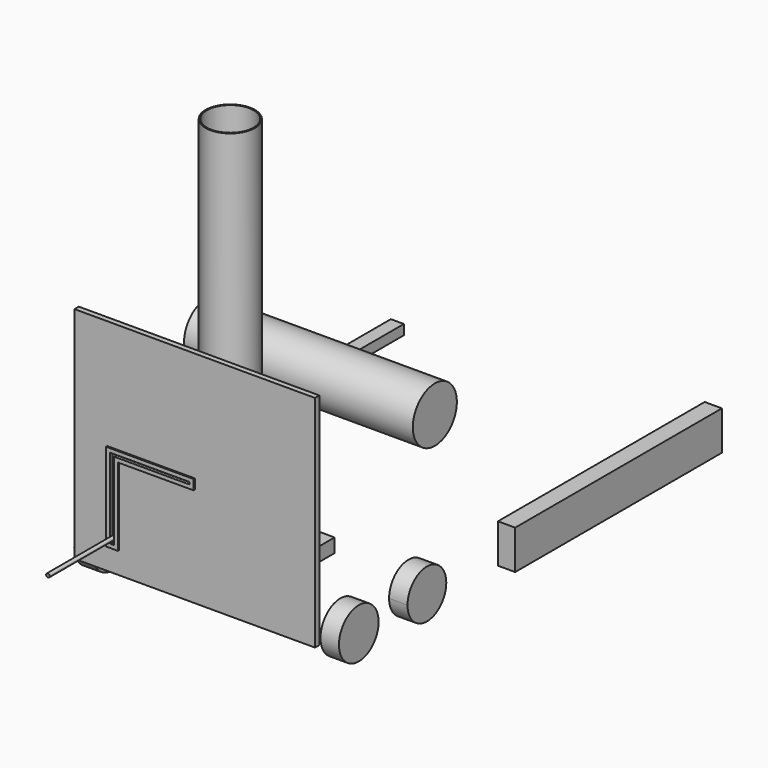
from build123d import *

# Parameters (mm, degrees)
F0_W      = 159.1055989265
F0_H      = 145.3896015882
F1_DEPTH  = 3.556
F6_R      = 18.1959049568
F7_DEPTH  = 151.384
F13_W     = 12.8093321323
F13_H     = 6.5816342831
F14_DEPTH = 36.068
F15_W     = 8.6199865751
F15_H     = 6.5816342831
F16_DEPTH = 170.942
F18_R     = 9.8295044078
F19_DEPTH = 25.4
F20_R     = 9.9402572171
F21_DEPTH = 1.016
F24_W     = 11.3966075535
F24_H     = 6.826877594
F25_DEPTH = 170.942
F26_R     = 16.3014838399
F27_DEPTH = 242.316
F28_R     = 15.4963138216
F29_DEPTH = 245.872
F31_DEPTH = 12.192
F33_DEPTH = 12.192
F34_W     = 34.9631672725
F34_H     = 28.9866179228
F35_DEPTH = 9.144
F36_T     = -2.54
F37_R     = 12.8059007853
F38_DEPTH = 3.048
F39_W     = 11.3966075535
F39_H     = 170.942
F40_DEPTH = 19.05
F43_W     = 50.1206144691
F43_H     = 6.5812724642
F44_DEPTH = 1.016
F45_T     = -2.54
F46_R     = 1.2184903026
F47_DEPTH = 54.864


# Not quite as in the source:
# - the program builds the solid bodies; features that only make, move or delete a surface that nothing else refers to are left out


with BuildPart() as f1:
    # F0 (on Front) → F1 (new body)
    with BuildSketch(Plane.XZ):
        Rectangle(F0_W, F0_H)
    extrude(amount=F1_DEPTH)

    # F18 (on face) → F19 (cut)
    with BuildSketch(Plane.XZ.offset(3.556)):
        with Locations((39.1956530511, -18.7452007085)):
            Circle(F18_R)
    extrude(amount=-F19_DEPTH, mode=Mode.SUBTRACT)

    # F20 (on face) → F21 (join)
    with BuildSketch(Plane.XZ.offset(3.556)):
        with Locations((39.1956530511, -18.7452007085)):
            Circle(F20_R)
    extrude(amount=-F21_DEPTH)

    # F43 (on face) → F44 (join)
    with BuildSketch(Plane.XZ.offset(3.556)):
        Polygon((-57.8088574111, 0), (-57.8088574111, -58.0925121903), (-50.1206144691, -58.0925121903), (-50.1206144691, -6.5812724642), (-50.1206144691, 0), align=None)
        with Locations((-25.0603072345, -3.2906362321)):
            Rectangle(F43_W, F43_H)
    extrude(amount=F44_DEPTH)

    # F45
    f45_openings = [f1.faces().sort_by_distance(p)[0] for p in [
        (-56.989309, -4.572, -29.046256),
    ]]
    offset(amount=F45_T, openings=f45_openings, kind=Kind.INTERSECTION)

    # F46 (on face) → F47 (join)
    with BuildSketch(Plane.XZ.offset(2.54)):
        with Locations((-54.0543831885, -52.2309578955)):
            Circle(F46_R)
    extrude(amount=F47_DEPTH)


with BuildPart() as f7:
    # F6 (on face) → F7 (new body)
    with BuildSketch(Plane.YZ.offset(74.9896243215)):
        with Locations((101.2156382203, 18.9172420651)):
            Circle(F6_R)
    extrude(amount=-F7_DEPTH)


with BuildPart() as f14:
    # F13 (on face) → F14 (new body)
    with BuildSketch(Plane.YZ.offset(-75.4310935736)):
        with Locations((120.5953339338, -69.4039836526)):
            Rectangle(F13_W, F13_H)
    extrude(amount=-F14_DEPTH)

    # F15 (on face) → F16 (join)
    with BuildSketch(Plane(origin=(0, 127, 0), x_dir=(-1, 0, 0), z_dir=(0, 1, 0))):
        with Locations((107.189100286, -69.4039836526)):
            Rectangle(F15_W, F15_H)
    extrude(amount=F16_DEPTH)


with BuildPart() as f25:
    # F24 (on face) → F25 (new body)
    with BuildSketch(Plane.XZ.offset(-127)):
        with Locations((101.8033205447, -69.2813619971)):
            Rectangle(F24_W, F24_H)
    extrude(amount=-F25_DEPTH)

    # F39 (on face) → F40 (join)
    with BuildSketch(Plane.XY.offset(-65.8679232001)):
        with Locations((101.8033205447, 212.471)):
            Rectangle(F39_W, F39_H)
    extrude(amount=F40_DEPTH)


with BuildPart() as f27:
    # F26 (on face) → F27 (new body)
    with BuildSketch(Plane.XY.offset(-44.9399761856)):
        with Locations((0, 25.7939305156)):
            Circle(F26_R)
    extrude(amount=F27_DEPTH)

    # F28 (on face) → F29 (cut)
    with BuildSketch(Plane.XY.offset(197.3760238144)):
        with Locations((0, 25.7939305156)):
            Circle(F28_R)
    extrude(amount=-F29_DEPTH, mode=Mode.SUBTRACT)


with BuildPart() as f31:
    # F30 (on face) → F31 (new body)
    with BuildSketch(Plane.YZ.offset(-75.4310935736)):
        with BuildLine():
            ThreePointArc((95.0685632255, -72.6948007941), (79.0285095572, -56.6547471259), (62.988455889, -72.6948007941))
            Line((62.988455889, -72.6948007941), (95.0685632255, -72.6948007941))
        make_face()
        with BuildLine():
            Line((95.0685632255, -72.6948007941), (62.988455889, -72.6948007941))
            ThreePointArc((62.988455889, -72.6948007941), (79.0285095572, -88.7348544623), (95.0685632255, -72.6948007941))
        make_face()
    extrude(amount=-F31_DEPTH)


with BuildPart() as f31b:
    # F30 (on face) → F31, piece 2 (new body)
    with BuildSketch(Plane.YZ.offset(-75.4310935736)):
        with BuildLine():
            Line((6.31843889, -72.6948007941), (38.4480318999, -72.6948007941))
            ThreePointArc((38.4480318999, -72.6948007941), (22.383235395, -56.6300042891), (6.31843889, -72.6948007941))
        make_face()
        with BuildLine():
            ThreePointArc((6.31843889, -72.6948007941), (22.383235395, -88.7595972991), (38.4480318999, -72.6948007941))
            Line((38.4480318999, -72.6948007941), (6.31843889, -72.6948007941))
        make_face()
    extrude(amount=-F31_DEPTH)


with BuildPart() as f33:
    # F32 (on face) → F33 (new body)
    with BuildSketch(Plane.YZ.offset(74.9896243215)):
        with BuildLine():
            Line((6.6852848444, -72.6948007941), (39.4695830132, -72.6948007941))
            ThreePointArc((39.4695830132, -72.6948007941), (23.0774339288, -56.3026517097), (6.6852848444, -72.6948007941))
        make_face()
        with BuildLine():
            ThreePointArc((6.6852848444, -72.6948007941), (23.0774339288, -89.0869498785), (39.4695830132, -72.6948007941))
            Line((39.4695830132, -72.6948007941), (6.6852848444, -72.6948007941))
        make_face()
    extrude(amount=F33_DEPTH)


with BuildPart() as f33b:
    # F32 (on face) → F33, piece 2 (new body)
    with BuildSketch(Plane.YZ.offset(74.9896243215)):
        with BuildLine():
            Line((95.4328895507, -72.6948007941), (63.3894979062, -72.6948007941))
            ThreePointArc((63.3894979062, -72.6948007941), (79.4111937284, -88.7164966163), (95.4328895507, -72.6948007941))
        make_face()
        with BuildLine():
            ThreePointArc((95.4328895507, -72.6948007941), (79.4111937284, -56.6731049719), (63.3894979062, -72.6948007941))
            Line((63.3894979062, -72.6948007941), (95.4328895507, -72.6948007941))
        make_face()
    extrude(amount=F33_DEPTH)


with BuildPart() as f35:
    # F34 (on face) → F35 (new body)
    with BuildSketch(Plane(origin=(0, 0, -72.6948007941), x_dir=(1, 0, 0), z_dir=(0, 0, -1))):
        with Locations((-7.0415311493, -84.5097303391)):
            Rectangle(F34_W, F34_H)
    extrude(amount=F35_DEPTH)

    # F36
    f36_openings = [f35.faces().sort_by_distance(p)[0] for p in [
        (-7.041531, 70.016421, -77.266801),
    ]]
    offset(amount=F36_T, openings=f36_openings)

    # F37 (on face) → F38 (join)
    with BuildSketch(Plane(origin=(0, 0, -75.2348007941), x_dir=(1, 0, 0), z_dir=(0, 0, -1))):
        with Locations((-6.2475237064, -84.7957953811)):
            Circle(F37_R)
    extrude(amount=F38_DEPTH)


solid = Compound([f1.part, f7.part, f14.part, f25.part, f27.part, f31.part, f31b.part, f33.part, f33b.part, f35.part])
